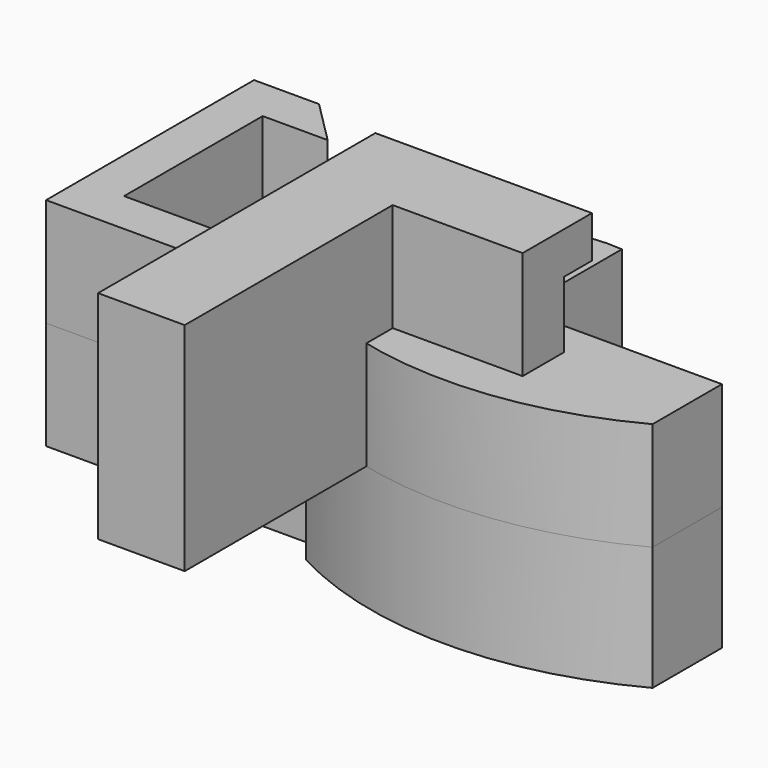
from build123d import *

# Parameters (mm, degrees)
F2_DEPTH = 28.6
F3_DEPTH = 25
F4_DEPTH = 25
F5_W     = 60
F5_H     = 50
F6_DEPTH = 20
F7_DEPTH = 50


with BuildPart() as f2:
    # F1 (on Top) → F2 (new body)
    with BuildSketch(Plane.XY):
        with BuildLine():
            Line((33.0262016572, 20), (33.0262016572, 49.8469781306))
            ThreePointArc((33.0262016572, 49.8469781306), (9.8851553538, 42.2574262856), (0, 20))
            Line((0, 20), (0, 0))
            ThreePointArc((0, 0), (40, -10), (80, 0))
            Line((80, 0), (80, 20))
            Line((80, 20), (33.0262016572, 20))
        make_face()
    extrude(amount=-F2_DEPTH)


with BuildPart() as f3:
    # F0 (on Top) → F3 (new body)
    with BuildSketch(Plane.XY):
        Polygon((-35, 50), (-45, 60), (-60, 60), (-60, 0), (0, 0), (-10, 10), (-50, 10), (-50, 50), align=None)
    extrude(amount=-F3_DEPTH)


with BuildPart() as f4:
    # F4 (new): a face of the model
    f4_faces = [f3.part.faces().sort_by_distance(p)[0] for p in [
        (-40.6, 54.4, 0),
    ]]
    extrude(f4_faces, amount=F4_DEPTH)


with BuildPart() as f4b:
    # F4#2 (new): a face of the model
    f4_2_faces = [f2.part.faces().sort_by_distance(p)[0] for p in [
        (34.2678216029, 13.6636139623, 0),
    ]]
    extrude(f4_2_faces, amount=F4_DEPTH)


with BuildPart() as f6:
    # F5 (on Right) → F6 (new body)
    with BuildSketch(Plane.YZ):
        with Locations((-30, 25)):
            Rectangle(F5_W, F5_H)
    extrude(amount=F6_DEPTH)

    # F5 (on Right) → F7 (join)
    with BuildSketch(Plane.YZ):
        Polygon((20, 50), (0, 50), (0, 0), (20, 0), (20, 10.3311939165), (12, 10.3311939165), (12, 40.3311939165), (20, 40.3311939165), align=None)
    extrude(amount=F7_DEPTH)


solid = Compound([f2.part, f3.part, f4.part, f4b.part, f6.part])
